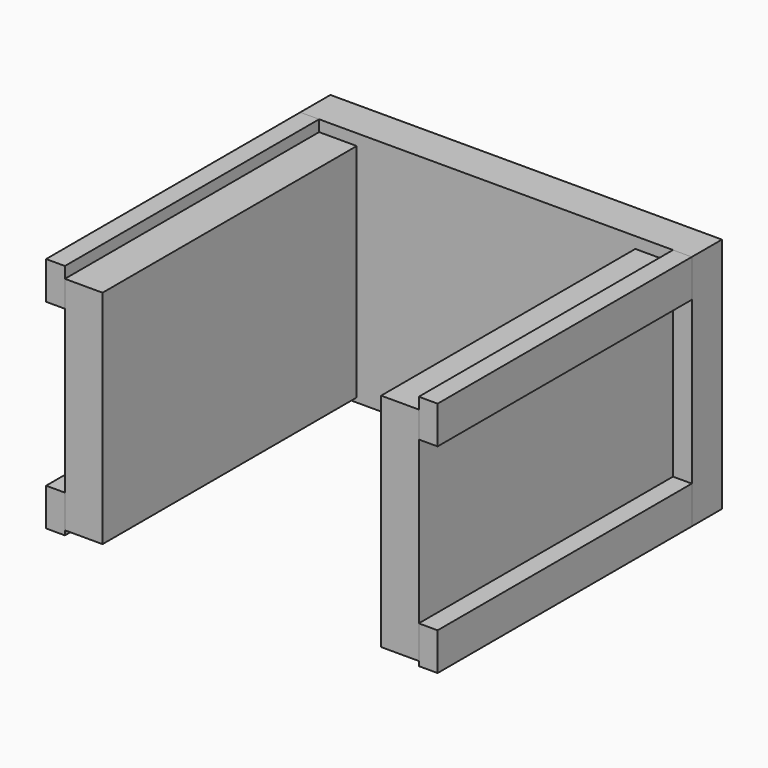
from build123d import *

# Parameters (mm, degrees)
F2_DEPTH = 422
F3_DEPTH = 422
F4_DEPTH = 422
F1_W     = 370
F1_H     = 294
F1_W_2   = 25
F1_H_2   = 215
F5_DEPTH = 50


# Not quite as in the source:
# - a feature names something its author has since deleted; it is built from what else it names


with BuildPart() as f2:
    # F1 (on Front) → F2 (new body)
    with BuildSketch(Plane.XZ):
        Polygon((-306.2545120716, 109.5745983869), (-306.2545120716, 144.5745983869), (-306.2545120716, 159.5745983869), (-331.2545120716, 159.5745983869), (-331.2545120716, 109.5745983869), align=None)
    extrude(amount=F2_DEPTH)


with BuildPart() as f2b:
    # F1 (on Front) → F2, piece 2 (new body)
    with BuildSketch(Plane.XZ):
        Polygon((163.7454879284, 159.5745983869), (163.7454879284, 144.5745983869), (163.7454879284, 109.5745983869), (188.7454879284, 109.5745983869), (188.7454879284, 159.5745983869), align=None)
    extrude(amount=F2_DEPTH)


with BuildPart() as f3:
    # F1 (on Front) → F3 (new body)
    with BuildSketch(Plane.XZ):
        Polygon((-306.2545120716, -149.4254016131), (-256.2545120716, -149.4254016131), (-256.2545120716, 144.5745983869), (-306.2545120716, 144.5745983869), (-306.2545120716, 109.5745983869), (-306.2545120716, -105.4254016131), align=None)
    extrude(amount=F3_DEPTH)


with BuildPart() as f3b:
    # F1 (on Front) → F3, piece 2 (new body)
    with BuildSketch(Plane.XZ):
        Polygon((113.7454879284, 144.5745983869), (113.7454879284, -149.4254016131), (163.7454879284, -149.4254016131), (163.7454879284, -105.4254016131), (163.7454879284, 109.5745983869), (163.7454879284, 144.5745983869), align=None)
    extrude(amount=F3_DEPTH)


with BuildPart() as f4:
    # F1 (on Front) → F4 (new body)
    with BuildSketch(Plane.XZ):
        Polygon((-306.2545120716, -155.4254016131), (-306.2545120716, -149.4254016131), (-306.2545120716, -105.4254016131), (-331.2545120716, -105.4254016131), (-331.2545120716, -155.4254016131), align=None)
    extrude(amount=F4_DEPTH)


with BuildPart() as f4b:
    # F1 (on Front) → F4, piece 2 (new body)
    with BuildSketch(Plane.XZ):
        Polygon((163.7454879284, -105.4254016131), (163.7454879284, -149.4254016131), (163.7454879284, -155.4254016131), (188.7454879284, -155.4254016131), (188.7454879284, -105.4254016131), align=None)
    extrude(amount=F4_DEPTH)


with BuildPart() as f5:
    # F1 (on Front) → F5 (new body)
    with BuildSketch(Plane.XZ):
        with Locations((-71.2545120716, -2.4254016131)):
            Rectangle(F1_W, F1_H)
        Polygon((-306.2545120716, -149.4254016131), (-256.2545120716, -149.4254016131), (-256.2545120716, 144.5745983869), (-306.2545120716, 144.5745983869), (-306.2545120716, 109.5745983869), (-306.2545120716, -105.4254016131), align=None)
        Polygon((113.7454879284, -149.4254016131), (-256.2545120716, -149.4254016131), (-306.2545120716, -149.4254016131), (-306.2545120716, -155.4254016131), (163.7454879284, -155.4254016131), (163.7454879284, -149.4254016131), align=None)
        Polygon((113.7454879284, 144.5745983869), (113.7454879284, -149.4254016131), (163.7454879284, -149.4254016131), (163.7454879284, -105.4254016131), (163.7454879284, 109.5745983869), (163.7454879284, 144.5745983869), align=None)
        Polygon((-306.2545120716, 144.5745983869), (-256.2545120716, 144.5745983869), (113.7454879284, 144.5745983869), (163.7454879284, 144.5745983869), (163.7454879284, 159.5745983869), (-306.2545120716, 159.5745983869), align=None)
        Polygon((-306.2545120716, -155.4254016131), (-306.2545120716, -149.4254016131), (-306.2545120716, -105.4254016131), (-331.2545120716, -105.4254016131), (-331.2545120716, -155.4254016131), align=None)
        Polygon((163.7454879284, -105.4254016131), (163.7454879284, -149.4254016131), (163.7454879284, -155.4254016131), (188.7454879284, -155.4254016131), (188.7454879284, -105.4254016131), align=None)
        Polygon((-306.2545120716, 109.5745983869), (-306.2545120716, 144.5745983869), (-306.2545120716, 159.5745983869), (-331.2545120716, 159.5745983869), (-331.2545120716, 109.5745983869), align=None)
        with Locations((-318.7545120716, 2.0745983869)):
            Rectangle(F1_W_2, F1_H_2)
        Polygon((163.7454879284, 159.5745983869), (163.7454879284, 144.5745983869), (163.7454879284, 109.5745983869), (188.7454879284, 109.5745983869), (188.7454879284, 159.5745983869), align=None)
        with Locations((176.2454879284, 2.0745983869)):
            Rectangle(F1_W_2, F1_H_2)
    extrude(amount=-F5_DEPTH)


solid = Compound([f2.part, f2b.part, f3.part, f3b.part, f4.part, f4b.part, f5.part])
